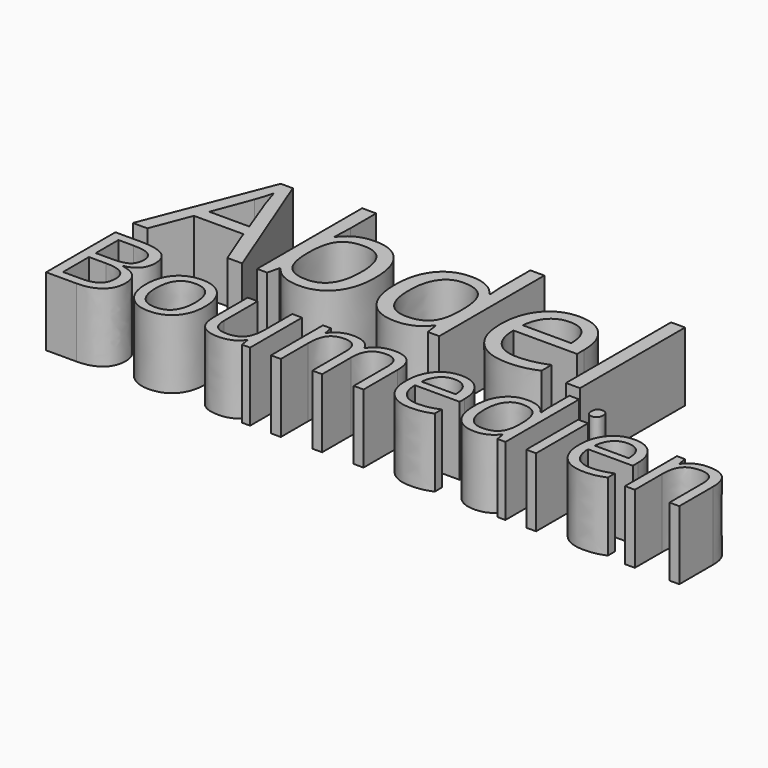
from build123d import *

# Parameters (mm, degrees)
F0_TEXT_SIZE   = 63.878560387
F0_TEXT_SIZE_2 = 44.8287309458
F1_DEPTH       = 25.4


# Not quite as in the source:
# - Text() gives the source's letters only with a copy of the font that has no kerning and outlines rounded to 1/6400 em; it was checked with that copy


with BuildPart() as f1:
    # F0 (on Top) → F1 (new body)
    with BuildSketch(Plane.XY):
        with Locations((-116.2769719958, -10.2565577254)):
            Text('Abdel', F0_TEXT_SIZE, font='Open Sans', text_align=(TextAlign.LEFT, TextAlign.BOTTOM))
        with Locations((-120.9811829031, -49.9266218394)):
            Text('Boumedien', F0_TEXT_SIZE_2, font='Open Sans', text_align=(TextAlign.LEFT, TextAlign.BOTTOM))
    extrude(amount=F1_DEPTH)


solid = f1.part
